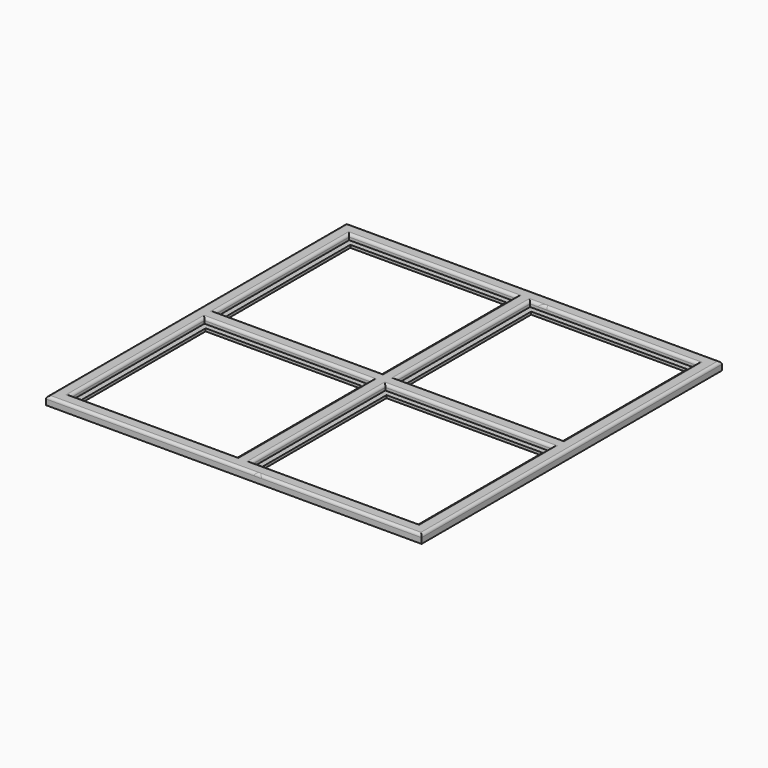
from build123d import *

# Parameters (mm, degrees)
F1_DEPTH = 3
F2_DEPTH = 1
F3_R     = 1
F3_2_R   = 1


# Not quite as in the source:
# - a feature names something its author has since deleted; it is built from what else it names


with BuildPart() as f1:
    # F0 (on Top) → F1 (new body)
    with BuildSketch(Plane.XY):
        with BuildLine():
            Line((-63.25, -34.2033516131), (-63.25, 26.5466483869))
            Line((-63.25, 26.5466483869), (-8.6602540378, 26.5466483869))
            ThreePointArc((-8.6602540378, 26.5466483869), (-9.6592582629, 28.9584579359), (-10, 31.5466483869))
            Line((-10, 31.5466483869), (-34.125, 31.5466483869))
            Line((-34.125, 31.5466483869), (-68.25, 31.5466483869))
            Line((-68.25, 31.5466483869), (-68.25, -36.7033516131))
            Line((-68.25, -36.7033516131), (0, -36.7033516131))
            Line((0, -36.7033516131), (0, 21.5466483869))
            ThreePointArc((0, 21.5466483869), (-1.2600429248, 21.6263514243), (-2.5, 21.8641900214))
            Line((-2.5, 21.8641900214), (-2.5, -34.2033516131))
            Line((-2.5, -34.2033516131), (-63.25, -34.2033516131))
        make_face()
        with BuildLine():
            ThreePointArc((-10, 31.5466483869), (-9.6592582629, 28.9584579359), (-8.6602540378, 26.5466483869))
            Line((-8.6602540378, 26.5466483869), (-5.4943754879, 26.5466483869))
            ThreePointArc((-5.4943754879, 26.5466483869), (-6.9283902407, 28.8660569086), (-7.4288735352, 31.5466483869))
            Line((-7.4288735352, 31.5466483869), (-10, 31.5466483869))
        make_face()
        with BuildLine():
            ThreePointArc((-7.4288735352, 31.5466483869), (-6.9283902407, 28.8660569086), (-5.4943754879, 26.5466483869))
            Line((-5.4943754879, 26.5466483869), (-2.5, 26.5466483869))
            Line((-2.5, 26.5466483869), (-2.5, 24.5510667812))
            ThreePointArc((-2.5, 24.5510667812), (-1.2686352802, 24.2268993115), (0, 24.1177748517))
            Line((0, 24.1177748517), (0, 31.5466483869))
            Line((0, 31.5466483869), (-7.4288735352, 31.5466483869))
        make_face()
        with BuildLine():
            ThreePointArc((0, 24.1177748517), (-1.2686352802, 24.2268993115), (-2.5, 24.5510667812))
            Line((-2.5, 24.5510667812), (-2.5, 21.8641900214))
            ThreePointArc((-2.5, 21.8641900214), (-1.2600429248, 21.6263514243), (0, 21.5466483869))
            Line((0, 21.5466483869), (0, 24.1177748517))
        make_face()
    extrude(amount=F1_DEPTH)

    # F0 (on Top) → F2 (join)
    with BuildSketch(Plane.XY):
        with BuildLine():
            Line((-8.6602540378, 26.5466483869), (-63.25, 26.5466483869))
            Line((-63.25, 26.5466483869), (-63.25, -34.2033516131))
            Line((-63.25, -34.2033516131), (-2.5, -34.2033516131))
            Line((-2.5, -34.2033516131), (-2.5, 21.8641900214))
            ThreePointArc((-2.5, 21.8641900214), (-3.5201478643, 22.1867039953), (-4.5, 22.6163628372))
            Line((-4.5, 22.6163628372), (-4.5, -32.2033516131))
            Line((-4.5, -32.2033516131), (-61.25, -32.2033516131))
            Line((-61.25, -32.2033516131), (-61.25, 24.5466483869))
            Line((-61.25, 24.5466483869), (-7.1414284285, 24.5466483869))
            ThreePointArc((-7.1414284285, 24.5466483869), (-7.9638741949, 25.4987803487), (-8.6602540378, 26.5466483869))
        make_face()
        with BuildLine():
            ThreePointArc((-10, 31.5466483869), (-9.6592582629, 28.9584579359), (-8.6602540378, 26.5466483869))
            Line((-8.6602540378, 26.5466483869), (-5.4943754879, 26.5466483869))
            ThreePointArc((-5.4943754879, 26.5466483869), (-6.9283902407, 28.8660569086), (-7.4288735352, 31.5466483869))
            Line((-7.4288735352, 31.5466483869), (-10, 31.5466483869))
        make_face()
        with BuildLine():
            Line((-5.4943754879, 26.5466483869), (-8.6602540378, 26.5466483869))
            ThreePointArc((-8.6602540378, 26.5466483869), (-7.9638741949, 25.4987803487), (-7.1414284285, 24.5466483869))
            Line((-7.1414284285, 24.5466483869), (-4.5, 24.5466483869))
            Line((-4.5, 24.5466483869), (-4.5, 22.6163628372))
            ThreePointArc((-4.5, 22.6163628372), (-3.5201478643, 22.1867039953), (-2.5, 21.8641900214))
            Line((-2.5, 21.8641900214), (-2.5, 24.5510667812))
            ThreePointArc((-2.5, 24.5510667812), (-4.1198417866, 25.364814868), (-5.4943754879, 26.5466483869))
        make_face()
        with BuildLine():
            Line((-2.5, 26.5466483869), (-5.4943754879, 26.5466483869))
            ThreePointArc((-5.4943754879, 26.5466483869), (-4.1198417866, 25.364814868), (-2.5, 24.5510667812))
            Line((-2.5, 24.5510667812), (-2.5, 26.5466483869))
        make_face()
    extrude(amount=F2_DEPTH)

    # F3
    f3_edges = [f1.edges().sort_by_distance(p)[0] for p in [
        (-32.875, 26.546648, 3),
        (-63.25, -3.828352, 3),
        (-32.875, -34.203352, 3),
        (-2.5, -3.828352, 3),
        (-34.125, 31.546648, 3),
        (-68.25, -2.578352, 3),
    ]]
    fillet(f3_edges, radius=F3_R)



with BuildPart() as f1b:
    # F0 (on Top) → F1, piece 2 (new body)
    with BuildSketch(Plane.XY):
        with BuildLine():
            ThreePointArc((8.6602540378, 26.5466483869), (9.6592582629, 28.9584579359), (10, 31.5466483869))
            Line((10, 31.5466483869), (7.4288735352, 31.5466483869))
            ThreePointArc((7.4288735352, 31.5466483869), (6.9283902407, 28.8660569086), (5.4943754879, 26.5466483869))
            Line((5.4943754879, 26.5466483869), (8.6602540378, 26.5466483869))
        make_face()
    extrude(amount=F1_DEPTH)

    # F0 (on Top) → F2, piece 2 (join)
    with BuildSketch(Plane.XY):
        with BuildLine():
            ThreePointArc((8.6602540378, 26.5466483869), (9.6592582629, 28.9584579359), (10, 31.5466483869))
            Line((10, 31.5466483869), (7.4288735352, 31.5466483869))
            ThreePointArc((7.4288735352, 31.5466483869), (6.9283902407, 28.8660569086), (5.4943754879, 26.5466483869))
            Line((5.4943754879, 26.5466483869), (8.6602540378, 26.5466483869))
        make_face()
    extrude(amount=F2_DEPTH)

    # F3#2
    f3_2_edges = [f1b.edges().sort_by_distance(p)[0] for p in [
        (9.659258, 28.958458, 3),
        (6.92839, 28.866057, 3),
        (7.077315, 26.546648, 3),
        (8.714437, 31.546648, 3),
    ]]
    fillet(f3_2_edges, radius=F3_2_R)


with BuildPart() as f1_1:
    add(f1.part)

    add(f1b.part)  # F4 merges F1b
    # F4: F1 across plane
    add(f1.part.mirror(Plane.YZ))

    # F5: F1 across face


with BuildPart() as f1_2:
    add(f1_1.part)
    add(f1_1.part.mirror(Plane(origin=(0, -36.7033516131, 1.4986605371), x_dir=(1, 0, 0), z_dir=(0, -1, 0))))


solid = f1_2.part
